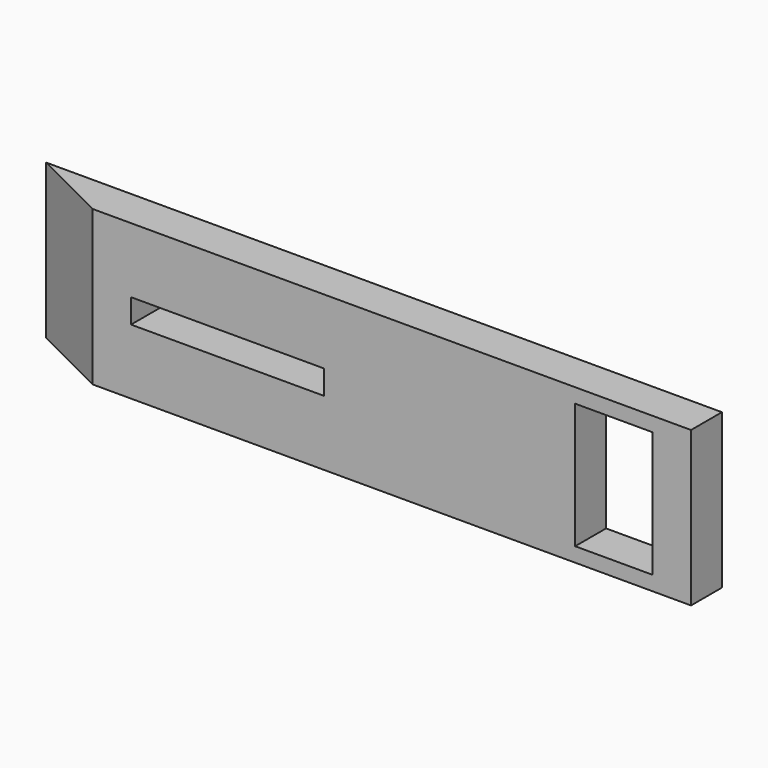
from build123d import *

# Parameters (mm, degrees)
F0_W     = 35
F0_H     = 8
F1_DEPTH = 2
F2_SIZE2 = 3.99999
F2_SIZE  = 1.99999
F3_W     = 4
F3_H     = 6.5
F4_DEPTH = 2
F5_W     = 10
F5_H     = 1.25
F6_DEPTH = 2


# Not quite as in the source:
# - a fillet or chamfer is up to 0.001 mm smaller than in the source, because OpenCascade refuses the exact size


with BuildPart() as f1:
    # F0 (on Front) → F1 (new body)
    with BuildSketch(Plane.XZ):
        with Locations((-17.5, 4)):
            Rectangle(F0_W, F0_H)
    extrude(amount=F1_DEPTH)

    # F2 (size 2 and 4 in the source; OpenCascade refuses exactly that, so slightly less here)
    f2_edges = [f1.edges().sort_by_distance(p)[0] for p in [
        (-35, -2, 4),
    ]]
    f2_side = f1.faces().sort_by_distance((-35, -1, 4))[0]
    chamfer(f2_edges, length=F2_SIZE, length2=F2_SIZE2, reference=f2_side)

    # F3 (on face) → F4 (cut)
    with BuildSketch(Plane.XZ.offset(2)):
        with Locations((-4, 4)):
            Rectangle(F3_W, F3_H)
    extrude(amount=-F4_DEPTH, mode=Mode.SUBTRACT)

    # F5 (on face) → F6 (cut)
    with BuildSketch(Plane.XZ.offset(2)):
        with Locations((-24, 4)):
            Rectangle(F5_W, F5_H)
    extrude(amount=-F6_DEPTH, mode=Mode.SUBTRACT)


solid = f1.part
